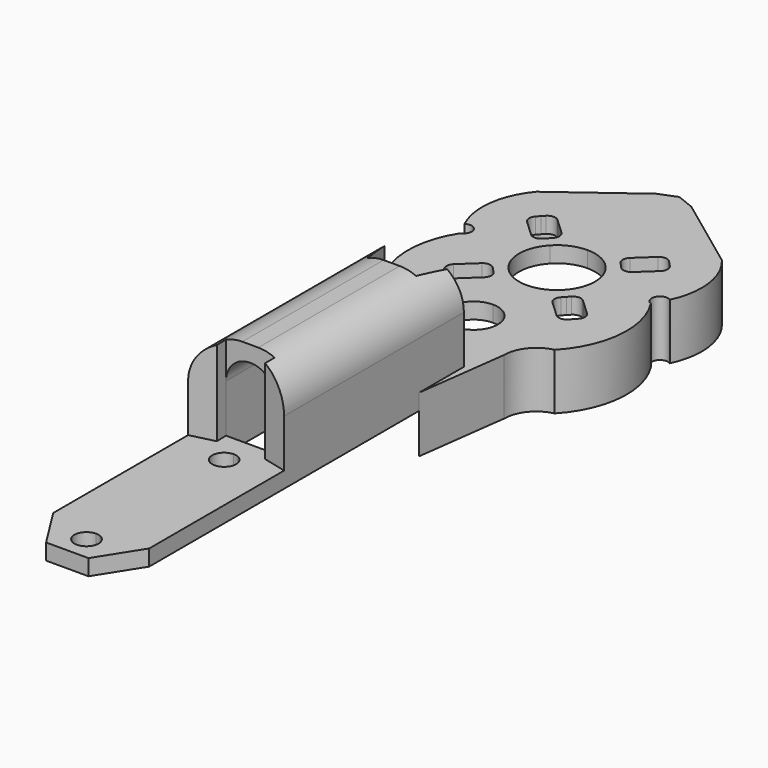
from build123d import *

# Parameters (mm, degrees)
F1_DEPTH     = 2
F0_W         = 3.0445663724
F0_H         = 3.2343552448
F0_H_2       = 18.850909546
F2_DEPTH     = 13
F3_DEPTH     = 11
F4_T4_DEPTH  = 22.0852647908
F4_T9_DEPTH  = 22.0852647908
F4_T15_DEPTH = 22.0852647908
F4_T20_DEPTH = 22.0852647908
F5_DEPTH     = 5
F6_T1_DEPTH  = 53.0795018189


# Not quite as in the source:
# - a fillet or chamfer that OpenCascade refuses, or shapes differently, is made with other operations: its cross-section is extruded or revolved along the edge and cut away or added


with BuildPart() as f1:
    # F0 (on Top) → F1 (new body)
    with BuildSketch(Plane.XY):
        with BuildLine():
            Line((0, -21.442663461), (0, -19.587084651))
            Line((0, -19.587084651), (-3, -20.329666324))
            Line((-3, -20.329666324), (-6, -21.0722479969))
            Line((-6, -21.0722479969), (-6, -42.1444959939))
            Line((-6, -42.1444959939), (-2.6490809396, -47.442663461))
            Line((-2.6490809396, -47.442663461), (0, -47.442663461))
            Line((0, -47.442663461), (0, -45.942663461))
            ThreePointArc((0, -45.942663461), (-1.5, -44.442663461), (0, -42.942663461))
            Line((0, -42.942663461), (0, -24.442663461))
            ThreePointArc((0, -24.442663461), (-1.5, -22.942663461), (0, -21.442663461))
        make_face()
        with BuildLine():
            Line((3.0445663724, -20.3406977144), (0, -19.587084651))
            Line((0, -19.587084651), (0, -21.442663461))
            ThreePointArc((0, -21.442663461), (1.0606601718, -21.8820032892), (1.5, -22.942663461))
            ThreePointArc((1.5, -22.942663461), (1.0606601718, -24.0033236327), (0, -24.442663461))
            Line((0, -24.442663461), (0, -42.942663461))
            ThreePointArc((0, -42.942663461), (1.0606601718, -43.3820032892), (1.5, -44.442663461))
            ThreePointArc((1.5, -44.442663461), (1.0606601718, -45.5033236327), (0, -45.942663461))
            Line((0, -45.942663461), (0, -47.442663461))
            Line((0, -47.442663461), (2.6490809396, -47.442663461))
            Line((2.6490809396, -47.442663461), (6, -42.1444959939))
            Line((6, -42.1444959939), (6, -21.0722479969))
            Line((6, -21.0722479969), (3.0445663724, -20.3406977144))
        make_face()
        Polygon((3.0445663724, -18.850909546), (0, -18.850909546), (0, -19.587084651), (3.0445663724, -20.3406977144), align=None)
        Polygon((0, -19.587084651), (0, -18.850909546), (-3.0445663724, -18.850909546), (-3, -20.329666324), align=None)
    extrude(amount=F1_DEPTH)



with BuildPart() as f1b:
    # F0 (on Top) → F1, piece 2 (new body)
    with BuildSketch(Plane.XY):
        with BuildLine():
            Line((-6, 7.0072538219), (-6, 11.414472945))
            ThreePointArc((-6, 11.414472945), (-7.0672827337, 14.6788128793), (-9.8568433896, 16.6821498424))
            ThreePointArc((-9.8568433896, 16.6821498424), (-12.1286787232, 22.0440734554), (-10.825092271, 27.7196459355))
            ThreePointArc((-10.825092271, 27.7196459355), (-9.8130602705, 30.3439953427), (-11.8637687892, 32.269096159))
            ThreePointArc((-11.8637687892, 32.269096159), (-12.0776575065, 35.9154722642), (-10.5480544763, 39.2324168906))
            Line((-10.5480544763, 39.2324168906), (-1.4462802792, 45.9774918854))
            Line((-1.4462802792, 45.9774918854), (0, 46.557336539))
            Line((0, 46.557336539), (1.4462802792, 45.9774918854))
            Line((1.4462802792, 45.9774918854), (10.5480544763, 39.2324168906))
            ThreePointArc((10.5480544763, 39.2324168906), (12.0776575065, 35.9154722642), (11.8637687892, 32.269096159))
            ThreePointArc((11.8637687892, 32.269096159), (9.8130602705, 30.3439953427), (10.825092271, 27.7196459355))
            ThreePointArc((10.825092271, 27.7196459355), (12.1286787232, 22.0440734554), (9.8568433896, 16.6821498424))
            ThreePointArc((9.8568433896, 16.6821498424), (7.0672827337, 14.6788128793), (6, 11.414472945))
            Line((6, 11.414472945), (6, 7.0072538219))
            Line((6, 7.0072538219), (6, 0))
            Line((6, 0), (7.5000002513, 11.414472945))
            ThreePointArc((7.5000002513, 11.414472945), (8.391991284, 13.9415584091), (10.6726818627, 15.3487753182))
            ThreePointArc((10.6726818627, 15.3487753182), (13.6200024271, 21.8800699646), (11.8968068959, 28.8352914154))
            ThreePointArc((11.8968068959, 28.8352914154), (11.3640087027, 30.251868892), (12.8284885302, 30.6337910005))
            ThreePointArc((12.8284885302, 30.6337910005), (13.635549564, 35.6633929404), (11.5888776878, 40.3280877233))
            Line((11.5888776878, 40.3280877233), (2.1839900136, 47.2977917949))
            Line((2.1839900136, 47.2977917949), (0, 48.173400037))
            Line((0, 48.173400037), (-2.1839900136, 47.2977917949))
            Line((-2.1839900136, 47.2977917949), (-11.5888776878, 40.3280877233))
            ThreePointArc((-11.5888776878, 40.3280877233), (-13.635549564, 35.6633929404), (-12.8284885302, 30.6337910005))
            ThreePointArc((-12.8284885302, 30.6337910005), (-11.3640087027, 30.251868892), (-11.8968068959, 28.8352914154))
            ThreePointArc((-11.8968068959, 28.8352914154), (-13.6200024271, 21.8800699646), (-10.6726818627, 15.3487753182))
            ThreePointArc((-10.6726818627, 15.3487753182), (-8.391991284, 13.9415584091), (-7.5000002513, 11.414472945))
            Line((-7.5000002513, 11.414472945), (-6, 0))
            Line((-6, 0), (-6, 7.0072538219))
        make_face()
        with BuildLine():
            Line((-6, 11.414472945), (0, 11.414472945))
            Line((0, 11.414472945), (0, 13.057336539))
            ThreePointArc((0, 13.057336539), (-3, 16.057336539), (0, 19.057336539))
            Line((0, 19.057336539), (0, 24.307336539))
            ThreePointArc((0, 24.307336539), (-1.892281439, 24.7005291121), (-3.4712866642, 25.8150119262))
            ThreePointArc((-3.4712866642, 25.8150119262), (-4.75, 29.057336539), (-3.4712866642, 32.2996611519))
            ThreePointArc((-3.4712866642, 32.2996611519), (-1.892281439, 33.414143966), (0, 33.807336539))
            Line((0, 33.807336539), (0, 46.557336539))
            Line((0, 46.557336539), (-1.4462802792, 45.9774918854))
            Line((-1.4462802792, 45.9774918854), (-10.5480544763, 39.2324168906))
            ThreePointArc((-10.5480544763, 39.2324168906), (-12.0776575065, 35.9154722642), (-11.8637687892, 32.269096159))
            ThreePointArc((-11.8637687892, 32.269096159), (-9.8130602705, 30.3439953427), (-10.825092271, 27.7196459355))
            ThreePointArc((-10.825092271, 27.7196459355), (-12.1286787232, 22.0440734554), (-9.8568433896, 16.6821498424))
            ThreePointArc((-9.8568433896, 16.6821498424), (-7.0672827337, 14.6788128793), (-6, 11.414472945))
        make_face()
        with BuildLine():
            Line((-4.9087797805, 25.1565185394), (-4.5674824529, 24.7911199432))
            Line((-4.5674824529, 24.7911199432), (-4.2261851252, 24.4257213469))
            ThreePointArc((-4.2261851252, 24.4257213469), (-3.9575633576, 23.7090423507), (-4.2743876623, 23.0123294991))
            Line((-4.2743876623, 23.0123294991), (-6.2840799416, 21.135194197))
            ThreePointArc((-6.2840799416, 21.135194197), (-7.0007589378, 20.8665724294), (-7.6974717894, 21.1833967341))
            Line((-7.6974717894, 21.1833967341), (-8.038769117, 21.5487953303))
            Line((-8.038769117, 21.5487953303), (-8.3800664447, 21.9141939265))
            ThreePointArc((-8.3800664447, 21.9141939265), (-8.6486882123, 22.6308729227), (-8.3318639076, 23.3275857743))
            Line((-8.3318639076, 23.3275857743), (-6.3221716283, 25.2047210765))
            ThreePointArc((-6.3221716283, 25.2047210765), (-5.6054926321, 25.4733428441), (-4.9087797805, 25.1565185394))
        make_face(mode=Mode.SUBTRACT)
        with BuildLine():
            Line((-4.2261851252, 33.6889517311), (-4.5674824529, 33.3235531349))
            Line((-4.5674824529, 33.3235531349), (-4.9087797805, 32.9581545387))
            ThreePointArc((-4.9087797805, 32.9581545387), (-5.6054926321, 32.641330234), (-6.3221716283, 32.9099520015))
            Line((-6.3221716283, 32.9099520015), (-8.3318639076, 34.7870873037))
            ThreePointArc((-8.3318639076, 34.7870873037), (-8.6486882123, 35.4838001553), (-8.3800664447, 36.2004791515))
            Line((-8.3800664447, 36.2004791515), (-8.038769117, 36.5658777478))
            Line((-8.038769117, 36.5658777478), (-7.6974717894, 36.931276344))
            ThreePointArc((-7.6974717894, 36.931276344), (-7.0007589378, 37.2481006487), (-6.2840799416, 36.9794788811))
            Line((-6.2840799416, 36.9794788811), (-4.2743876623, 35.1023435789))
            ThreePointArc((-4.2743876623, 35.1023435789), (-3.9575633576, 34.4056307273), (-4.2261851252, 33.6889517311))
        make_face(mode=Mode.SUBTRACT)
        with BuildLine():
            Line((0, 13.057336539), (0, 11.414472945))
            Line((0, 11.414472945), (6, 11.414472945))
            ThreePointArc((6, 11.414472945), (7.0672827337, 14.6788128793), (9.8568433896, 16.6821498424))
            ThreePointArc((9.8568433896, 16.6821498424), (12.1286787232, 22.0440734554), (10.825092271, 27.7196459355))
            ThreePointArc((10.825092271, 27.7196459355), (9.8130602705, 30.3439953427), (11.8637687892, 32.269096159))
            ThreePointArc((11.8637687892, 32.269096159), (12.0776575065, 35.9154722642), (10.5480544763, 39.2324168906))
            Line((10.5480544763, 39.2324168906), (1.4462802792, 45.9774918854))
            Line((1.4462802792, 45.9774918854), (0, 46.557336539))
            Line((0, 46.557336539), (0, 33.807336539))
            ThreePointArc((0, 33.807336539), (1.892281439, 33.414143966), (3.4712866642, 32.2996611519))
            ThreePointArc((3.4712866642, 32.2996611519), (4.4187731134, 30.8000195775), (4.75, 29.057336539))
            ThreePointArc((4.75, 29.057336539), (4.4187731134, 27.3146535006), (3.4712866642, 25.8150119262))
            ThreePointArc((3.4712866642, 25.8150119262), (1.892281439, 24.7005291121), (0, 24.307336539))
            Line((0, 24.307336539), (0, 19.057336539))
            ThreePointArc((0, 19.057336539), (2.1213203436, 18.1786568826), (3, 16.057336539))
            ThreePointArc((3, 16.057336539), (2.1213203436, 13.9360161955), (0, 13.057336539))
        make_face()
        with BuildLine():
            Line((4.2261851252, 24.4257213469), (4.5674824529, 24.7911199432))
            Line((4.5674824529, 24.7911199432), (4.9087797805, 25.1565185394))
            ThreePointArc((4.9087797805, 25.1565185394), (5.6054926321, 25.4733428441), (6.3221716283, 25.2047210765))
            Line((6.3221716283, 25.2047210765), (8.3318639076, 23.3275857743))
            ThreePointArc((8.3318639076, 23.3275857743), (8.6486882123, 22.6308729227), (8.3800664447, 21.9141939265))
            Line((8.3800664447, 21.9141939265), (8.038769117, 21.5487953303))
            Line((8.038769117, 21.5487953303), (7.6974717894, 21.1833967341))
            ThreePointArc((7.6974717894, 21.1833967341), (7.0007589378, 20.8665724294), (6.2840799416, 21.135194197))
            Line((6.2840799416, 21.135194197), (4.2743876623, 23.0123294991))
            ThreePointArc((4.2743876623, 23.0123294991), (3.9575633576, 23.7090423507), (4.2261851252, 24.4257213469))
        make_face(mode=Mode.SUBTRACT)
        with BuildLine():
            Line((4.9087797805, 32.9581545387), (4.5674824529, 33.3235531349))
            Line((4.5674824529, 33.3235531349), (4.2261851252, 33.6889517311))
            ThreePointArc((4.2261851252, 33.6889517311), (3.9575633576, 34.4056307273), (4.2743876623, 35.1023435789))
            Line((4.2743876623, 35.1023435789), (6.2840799416, 36.9794788811))
            ThreePointArc((6.2840799416, 36.9794788811), (7.0007589378, 37.2481006487), (7.6974717894, 36.931276344))
            Line((7.6974717894, 36.931276344), (8.038769117, 36.5658777478))
            Line((8.038769117, 36.5658777478), (8.3800664447, 36.2004791515))
            ThreePointArc((8.3800664447, 36.2004791515), (8.6486882123, 35.4838001553), (8.3318639076, 34.7870873037))
            Line((8.3318639076, 34.7870873037), (6.3221716283, 32.9099520015))
            ThreePointArc((6.3221716283, 32.9099520015), (5.6054926321, 32.641330234), (4.9087797805, 32.9581545387))
        make_face(mode=Mode.SUBTRACT)
        Polygon((0, 11.414472945), (0, 7.0072538219), (3.9053543005, 7.0072538219), (6, 7.0072538219), (6, 11.414472945), align=None)
        Polygon((-3.9053543005, 7.0072538219), (0, 7.0072538219), (0, 11.414472945), (-6, 11.414472945), (-6, 7.0072538219), align=None)
        Polygon((0, 3.2343552448), (0, 7.0072538219), (-3.9053543005, 7.0072538219), (-3.0445663724, 3.2343552448), align=None)
        Polygon((3.9053543005, 7.0072538219), (0, 7.0072538219), (0, 3.2343552448), (3.0445663724, 3.2343552448), align=None)
    extrude(amount=F1_DEPTH)


with BuildPart() as f1_1:
    add(f1.part)

    add(f1b.part)  # F2 merges F1b
    # F0 (on Top) → F2 (join)
    with BuildSketch(Plane.XY):
        with Locations((1.5222831862, 1.6171776224)):
            Rectangle(F0_W, F0_H)
        Polygon((-3.0445663724, 3.2343552448), (-3.9053543005, 7.0072538219), (-6, 7.0072538219), (-6, 0), (-6, -21.0722479969), (-3, -20.329666324), (-3.0445663724, -18.850909546), align=None)
        with Locations((1.5222831862, -9.425454773)):
            Rectangle(F0_W, F0_H_2)
        Polygon((0, 0), (0, 3.2343552448), (-3.0445663724, 3.2343552448), (-3.0445663724, -18.850909546), (0, -18.850909546), align=None)
        Polygon((6, 0), (3.0445663724, 0), (3.0445663724, -18.850909546), (3.0445663724, -20.3406977144), (6, -21.0722479969), align=None)
        Polygon((6, 7.0072538219), (3.9053543005, 7.0072538219), (3.0445663724, 3.2343552448), (3.0445663724, 0), (6, 0), align=None)
    extrude(amount=F2_DEPTH)

    # F0 (on Top) → F3 (cut)
    with BuildSketch(Plane.XY):
        Polygon((0, 0), (0, 3.2343552448), (-3.0445663724, 3.2343552448), (-3.0445663724, -18.850909546), (0, -18.850909546), align=None)
        with Locations((1.5222831862, -9.425454773)):
            Rectangle(F0_W, F0_H_2)
        with Locations((1.5222831862, 1.6171776224)):
            Rectangle(F0_W, F0_H)
    extrude(amount=F3_DEPTH, mode=Mode.SUBTRACT)

    # F4: fillet of radius 3 on 2 edges, made by hand


with BuildPart() as f4_tool2:
    # F4_s3 → F4_t4 (new body)
    with BuildSketch(Plane.XZ.offset(-3.2343552448)):
        with BuildLine():
            ThreePointArc((-3.0445663724, 8), (-2.165886716, 10.1213203436), (-0.0445663724, 11))
            Line((-0.0445663724, 11), (-3.0445663724, 11))
            Line((-3.0445663724, 11), (-3.0445663724, 8))
        make_face()
    extrude(amount=F4_T4_DEPTH)

    split(bisect_by=Plane(origin=(-2.1925209423, -0.5002243025, 0), x_dir=(0, 0, 1), z_dir=(0.9749476162, 0.2224345875, 0)), keep=Keep.TOP)


with BuildPart() as f1_2:
    add(f1_1.part)

    # F4_t1: union F4_tool2
    add(f4_tool2.part)


with BuildPart() as f4_tool7:
    # F4_s8 → F4_t9 (new body)
    with BuildSketch(Plane.XZ.offset(-3.2343552448)):
        with BuildLine():
            ThreePointArc((-3.0445663724, 8), (-2.165886716, 10.1213203436), (-0.0445663724, 11))
            Line((-0.0445663724, 11), (-3.0445663724, 11))
            Line((-3.0445663724, 11), (-3.0445663724, 8))
        make_face()
    extrude(amount=F4_T9_DEPTH)

    split(bisect_by=Plane(origin=(-2.1925209423, -0.5002243025, 0), x_dir=(0, 0, 1), z_dir=(-0.9749476162, -0.2224345875, 0)), keep=Keep.TOP)

    split(bisect_by=Plane(origin=(-3.6094116269, -0.1087794728, 0), x_dir=(0, 0, 1), z_dir=(0.9995461677, 0.0301240525, 0)), keep=Keep.TOP)


with BuildPart() as f1_3:
    add(f1_2.part)

    # F4_t6: union F4_tool7
    add(f4_tool7.part)


with BuildPart() as f4_tool13:
    # F4_s14 → F4_t15 (new body)
    with BuildSketch(Plane.XZ.offset(18.850909546)):
        with BuildLine():
            ThreePointArc((3.0445663724, 8), (2.165886716, 10.1213203436), (0.0445663724, 11))
            Line((0.0445663724, 11), (3.0445663724, 11))
            Line((3.0445663724, 11), (3.0445663724, 8))
        make_face()
    extrude(amount=-F4_T15_DEPTH)

    split(bisect_by=Plane(origin=(2.1925209423, -0.5002243025, 0), x_dir=(0, 0, 1), z_dir=(0.9749476162, -0.2224345875, 0)), keep=Keep.TOP)


with BuildPart() as f1_4:
    add(f1_3.part)

    # F4_t12: union F4_tool13
    add(f4_tool13.part)


with BuildPart() as f4_tool18:
    # F4_s19 → F4_t20 (new body)
    with BuildSketch(Plane.XZ.offset(18.850909546)):
        with BuildLine():
            ThreePointArc((3.0445663724, 8), (2.165886716, 10.1213203436), (0.0445663724, 11))
            Line((0.0445663724, 11), (3.0445663724, 11))
            Line((3.0445663724, 11), (3.0445663724, 8))
        make_face()
    extrude(amount=-F4_T20_DEPTH)

    split(bisect_by=Plane(origin=(2.1925209423, -0.5002243025, 0), x_dir=(0, 0, 1), z_dir=(-0.9749476162, 0.2224345875, 0)), keep=Keep.TOP)


with BuildPart() as f1_5:
    add(f1_4.part)

    # F4_t17: union F4_tool18
    add(f4_tool18.part)

    # F0 (on Top) → F5 (join)
    with BuildSketch(Plane.XY):
        with BuildLine():
            Line((-6, 7.0072538219), (-6, 11.414472945))
            ThreePointArc((-6, 11.414472945), (-7.0672827337, 14.6788128793), (-9.8568433896, 16.6821498424))
            ThreePointArc((-9.8568433896, 16.6821498424), (-12.1286787232, 22.0440734554), (-10.825092271, 27.7196459355))
            ThreePointArc((-10.825092271, 27.7196459355), (-9.8130602705, 30.3439953427), (-11.8637687892, 32.269096159))
            ThreePointArc((-11.8637687892, 32.269096159), (-12.0776575065, 35.9154722642), (-10.5480544763, 39.2324168906))
            Line((-10.5480544763, 39.2324168906), (-1.4462802792, 45.9774918854))
            Line((-1.4462802792, 45.9774918854), (0, 46.557336539))
            Line((0, 46.557336539), (1.4462802792, 45.9774918854))
            Line((1.4462802792, 45.9774918854), (10.5480544763, 39.2324168906))
            ThreePointArc((10.5480544763, 39.2324168906), (12.0776575065, 35.9154722642), (11.8637687892, 32.269096159))
            ThreePointArc((11.8637687892, 32.269096159), (9.8130602705, 30.3439953427), (10.825092271, 27.7196459355))
            ThreePointArc((10.825092271, 27.7196459355), (12.1286787232, 22.0440734554), (9.8568433896, 16.6821498424))
            ThreePointArc((9.8568433896, 16.6821498424), (7.0672827337, 14.6788128793), (6, 11.414472945))
            Line((6, 11.414472945), (6, 7.0072538219))
            Line((6, 7.0072538219), (6, 0))
            Line((6, 0), (7.5000002513, 11.414472945))
            ThreePointArc((7.5000002513, 11.414472945), (8.391991284, 13.9415584091), (10.6726818627, 15.3487753182))
            ThreePointArc((10.6726818627, 15.3487753182), (13.6200024271, 21.8800699646), (11.8968068959, 28.8352914154))
            ThreePointArc((11.8968068959, 28.8352914154), (11.3640087027, 30.251868892), (12.8284885302, 30.6337910005))
            ThreePointArc((12.8284885302, 30.6337910005), (13.635549564, 35.6633929404), (11.5888776878, 40.3280877233))
            Line((11.5888776878, 40.3280877233), (2.1839900136, 47.2977917949))
            Line((2.1839900136, 47.2977917949), (0, 48.173400037))
            Line((0, 48.173400037), (-2.1839900136, 47.2977917949))
            Line((-2.1839900136, 47.2977917949), (-11.5888776878, 40.3280877233))
            ThreePointArc((-11.5888776878, 40.3280877233), (-13.635549564, 35.6633929404), (-12.8284885302, 30.6337910005))
            ThreePointArc((-12.8284885302, 30.6337910005), (-11.3640087027, 30.251868892), (-11.8968068959, 28.8352914154))
            ThreePointArc((-11.8968068959, 28.8352914154), (-13.6200024271, 21.8800699646), (-10.6726818627, 15.3487753182))
            ThreePointArc((-10.6726818627, 15.3487753182), (-8.391991284, 13.9415584091), (-7.5000002513, 11.414472945))
            Line((-7.5000002513, 11.414472945), (-6, 0))
            Line((-6, 0), (-6, 7.0072538219))
        make_face()
    extrude(amount=-F5_DEPTH)

    # F6: fillet of radius 5 on 3 edges, made by hand

    # F6_s2 → F6_t1 (cut)
    with BuildSketch(Plane.XZ.offset(-19.5072538219)):
        with BuildLine():
            ThreePointArc((6, 8), (4.5355339059, 11.5355339059), (1, 13))
            Line((1, 13), (6, 13))
            Line((6, 13), (6, 8))
        make_face()
        with BuildLine():
            ThreePointArc((-6, 8), (-4.5355339059, 11.5355339059), (-1, 13))
            Line((-1, 13), (-6, 13))
            Line((-6, 13), (-6, 8))
        make_face()
    extrude(amount=F6_T1_DEPTH, mode=Mode.SUBTRACT)


solid = f1_5.part
